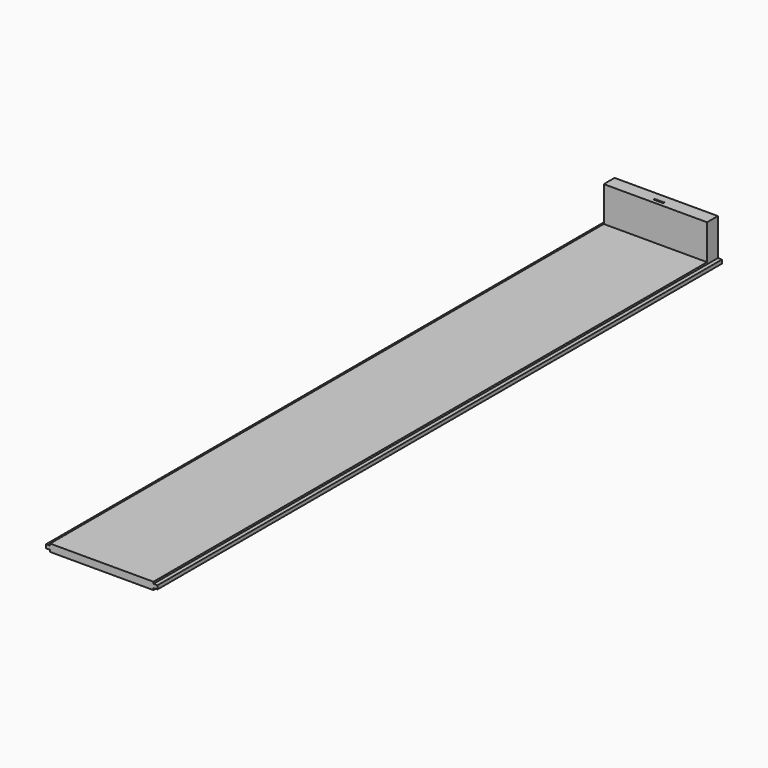
from build123d import *

# Parameters (mm, degrees)
F3_W        = 6.5772142261
F3_H        = 0.2320141066
F3_H_2      = 0.1190071926
F3_W_2      = 0.2564042807
F4_DEPTH    = 44.915836
F0_W        = 6.5772142261
F0_H        = 0.8592968807
F1_DEPTH    = 2.2352
F5_W        = 0.5953289354
F5_H        = 0.37034665
F6_DEPTH    = 0.03048
F7_T4_DEPTH = 1.9017438932
F2_SIZE     = 0.0254


# Not quite as in the source:
# - a fillet or chamfer that OpenCascade refuses, or shapes differently, is made with other operations: its cross-section is extruded or revolved along the edge and cut away or added


with BuildPart() as f4:
    # F3 (on Front) → F4 (new body)
    with BuildSketch(Plane.XZ):
        with Locations((0.5059395559, 0.0361560378)):
            Rectangle(F3_W, F3_H)
        with Locations((0.5059395559, 0.2116666874)):
            Rectangle(F3_W, F3_H_2)
        with Locations((0.5059395559, -0.1393546117)):
            Rectangle(F3_W, F3_H_2)
        with Locations((-2.9108696975, 0.0361560378)):
            Rectangle(F3_W_2, F3_H)
        with Locations((3.9227488093, 0.0361560378)):
            Rectangle(F3_W_2, F3_H)
    extrude(amount=F4_DEPTH)

    # F0 (on face) → F1 (join)
    with BuildSketch(Plane.XY.offset(0.2711702837)):
        with Locations((0.5059395559, -0.4296487314)):
            Rectangle(F0_W, F0_H)
    extrude(amount=F1_DEPTH)

    # F5 (on face) → F6 (join)
    with BuildSketch(Plane.XY.offset(2.5063702837)):
        with Locations((0.5059395559, -0.4296485859)):
            Rectangle(F5_W, F5_H)
    extrude(amount=F6_DEPTH)

    # F7: chamfer of 0.254 on 1 edges, made by hand


with BuildPart() as f7_tool2:
    # F7_s3 → F7_t4 (new body)
    with BuildSketch(Plane.YZ.offset(1.4568115025)):
        Polygon((-0.2444752608, 2.2828502837), (-0.4984752608, 2.5368502837), (-0.2444752608, 2.5368502837), align=None)
    extrude(amount=-F7_T4_DEPTH)

    split(bisect_by=Plane.XY.offset(2.5063702837), keep=Keep.TOP)


with BuildPart() as f4_1:
    add(f4.part)

    # F7_t1: cut F7_tool2
    add(f7_tool2.part, mode=Mode.SUBTRACT)

    # F2
    f2_edges = [f4_1.edges().sort_by_distance(p)[0] for p in [
        (0.50594, -0.614822, 2.53685),
    ]]
    chamfer(f2_edges, length=F2_SIZE)


solid = f4_1.part
